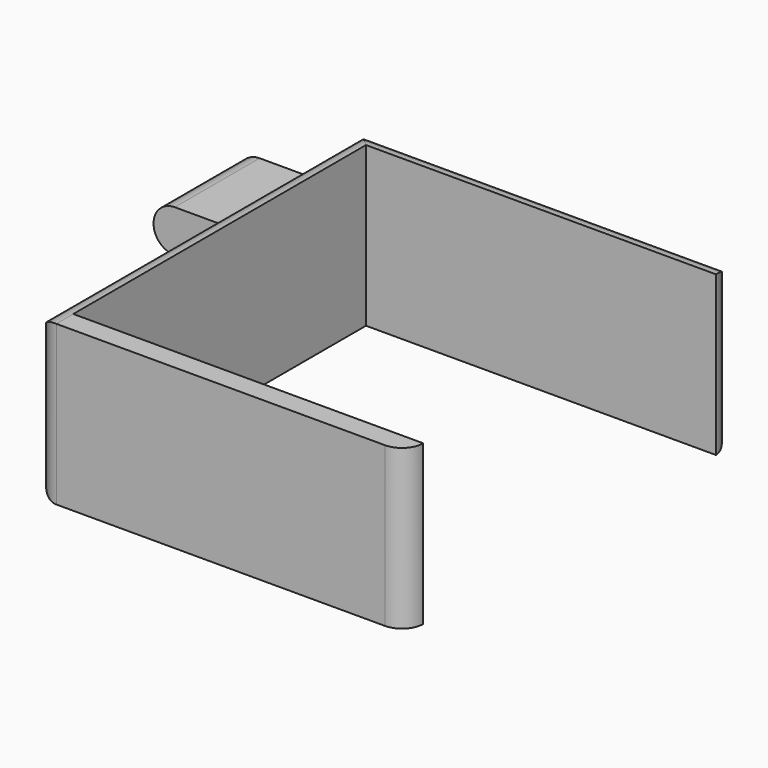
from build123d import *

# Parameters (mm, degrees)
F1_DEPTH    = 7.5
F2_R        = 1.99999
F4_DEPTH    = 5
F5_DEPTH    = 5
F6_T1_DEPTH = 20


# Not quite as in the source:
# - a fillet or chamfer that OpenCascade refuses, or shapes differently, is made with other operations: its cross-section is extruded or revolved along the edge and cut away or added
# - a fillet or chamfer is up to 0.001 mm smaller than in the source, because OpenCascade refuses the exact size


with BuildPart() as f1:
    # F0 (on Top) → F1 (new body, symmetric)
    with BuildSketch(Plane.XY):
        Polygon((29.4704200836, 8.5355388032), (29.4704200836, 10.5355388032), (-5.5295799164, 10.5355388032), (-5.5295799164, -27.9644611968), (29.4704200836, -27.9644611968), (29.4704200836, -25.9644611968), (27.4704200836, -25.9644611968), (-3.5295799164, -25.9644611968), (-3.5295799164, 8.5355388032), (27.4704200836, 8.5355388032), align=None)
    extrude(amount=F1_DEPTH, both=True)

    # F2 (radius 2 in the source; OpenCascade refuses exactly that, so slightly less here)
    f2_edges = [f1.edges().sort_by_distance(p)[0] for p in [
        (11.97042, 10.535539, 7.5),
        (11.97042, 10.535539, -7.5),
        (-5.52958, -8.714461, 7.5),
        (29.47042, -27.964461, 0),
        (-5.52958, -27.964461, 0),
        (29.47042, 10.535539, 0),
        (-5.52958, -8.714461, -7.5),
    ]]
    fillet(f2_edges, radius=F2_R)

    # F3 (on Front) → F4 (join, symmetric)
    with BuildSketch(Plane.XZ):
        with BuildLine():
            ThreePointArc((-11.7295799164, 1.7323087668), (-9.1295799164, 4.000441756), (-6.5295799164, 1.7323087668))
            Line((-6.5295799164, 1.7323087668), (-6.5295799164, -1.7323087668))
            ThreePointArc((-6.5295799164, -1.7323087668), (-9.1295799164, -4.000441756), (-11.7295799164, -1.7323087668))
            Line((-11.7295799164, -1.7323087668), (-11.7295799164, -1.5))
            Line((-11.7295799164, -1.5), (-12.7295799164, -1.5))
            Line((-12.7295799164, -1.5), (-12.7295799164, -5.500441756))
            Line((-12.7295799164, -5.500441756), (-5.5295799164, -5.500441756))
            Line((-5.5295799164, -5.500441756), (-5.5295799164, 5.500441756))
            Line((-5.5295799164, 5.500441756), (-12.7295799164, 5.500441756))
            Line((-12.7295799164, 5.500441756), (-12.7295799164, 1.5))
            Line((-12.7295799164, 1.5), (-11.7295799164, 1.5))
            Line((-11.7295799164, 1.5), (-11.7295799164, 1.7323087668))
        make_face()
    extrude(amount=F4_DEPTH, both=True)

    # F3 (on Front) → F5 (join)
    with BuildSketch(Plane.XZ):
        with BuildLine():
            Line((-6.5295799164, -1.7323087668), (-6.5295799164, 1.7323087668))
            ThreePointArc((-6.5295799164, 1.7323087668), (-9.1295799164, 4.000441756), (-11.7295799164, 1.7323087668))
            Line((-11.7295799164, 1.7323087668), (-11.7295799164, 1.5))
            Line((-11.7295799164, 1.5), (-10.5992737621, 1.5))
            ThreePointArc((-10.5992737621, 1.5), (-8.3160558159, 1.9360213165), (-7.0295799164, 0))
            ThreePointArc((-7.0295799164, 0), (-8.3160558159, -1.9360213165), (-10.5992737621, -1.5))
            Line((-10.5992737621, -1.5), (-11.7295799164, -1.5))
            Line((-11.7295799164, -1.5), (-11.7295799164, -1.7323087668))
            ThreePointArc((-11.7295799164, -1.7323087668), (-9.1295799164, -4.000441756), (-6.5295799164, -1.7323087668))
        make_face()
    extrude(amount=F5_DEPTH)

    # F6: fillet of radius 2 on 4 edges, made by hand

    # F6_s2 → F6_t1 (cut)
    with BuildSketch(Plane.XZ.offset(-10)):
        with BuildLine():
            ThreePointArc((-12.7295799164, 3.500441756), (-12.1437934788, 4.9146553183), (-10.7295799164, 5.500441756))
            Line((-10.7295799164, 5.500441756), (-12.7295799164, 5.500441756))
            Line((-12.7295799164, 5.500441756), (-12.7295799164, 3.500441756))
        make_face()
        with BuildLine():
            ThreePointArc((-10.7295799164, -5.500441756), (-12.1437934788, -4.9146553183), (-12.7295799164, -3.500441756))
            Line((-12.7295799164, -3.500441756), (-12.7295799164, -5.500441756))
            Line((-12.7295799164, -5.500441756), (-10.7295799164, -5.500441756))
        make_face()
        with BuildLine():
            ThreePointArc((-10.7295799164, 1.5), (-12.1437934788, 2.0857864376), (-12.7295799164, 3.5))
            Line((-12.7295799164, 3.5), (-12.7295799164, 1.5))
            Line((-12.7295799164, 1.5), (-10.7295799164, 1.5))
        make_face()
        with BuildLine():
            ThreePointArc((-10.7295799164, -1.5), (-12.1437934788, -2.0857864376), (-12.7295799164, -3.5))
            Line((-12.7295799164, -3.5), (-12.7295799164, -1.5))
            Line((-12.7295799164, -1.5), (-10.7295799164, -1.5))
        make_face()
    extrude(amount=F6_T1_DEPTH, mode=Mode.SUBTRACT)


solid = f1.part
